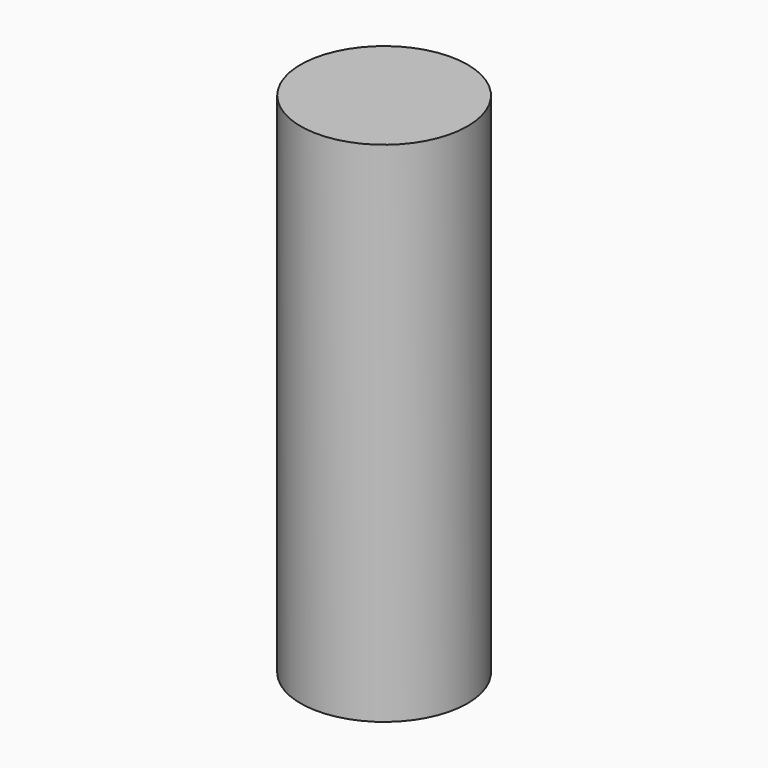
from build123d import *

# Parameters (mm, degrees)
F2_R     = 4.1075206271
F3_DEPTH = 25


# Not quite as in the source:
# - the program builds the solid bodies; features that only make, move or delete a surface that nothing else refers to are left out


with BuildPart() as f3:
    # F2 (on face) → F3 (new body)
    with BuildSketch(Plane.XY):
        Circle(F2_R)
    extrude(amount=F3_DEPTH)


solid = f3.part
